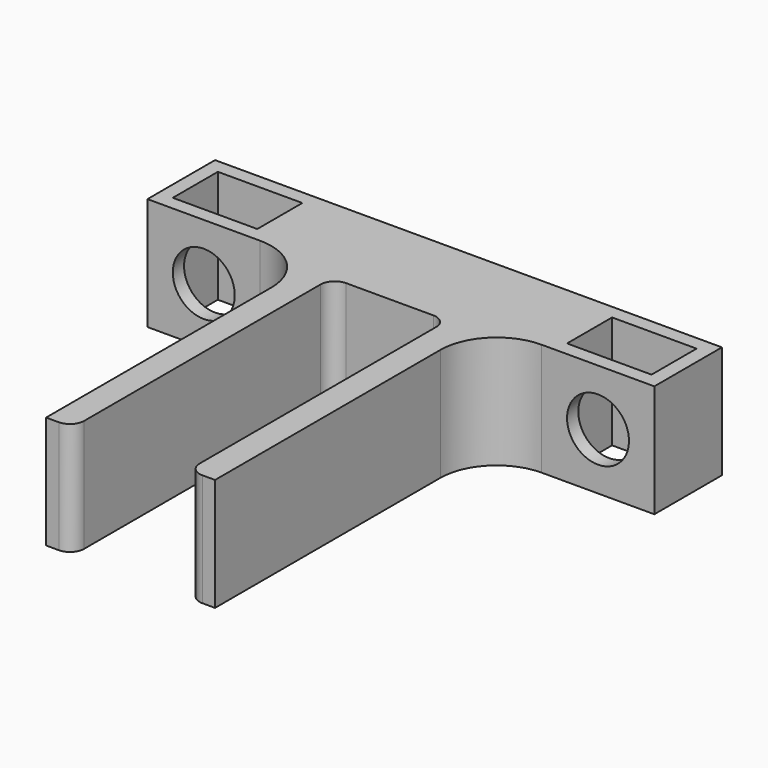
from build123d import *

# Parameters (mm, degrees)
F0_W         = 180
F0_H         = 40
F1_DEPTH     = 15
F2_W         = 60
F2_H         = 40
F3_DEPTH     = 120
F4_W         = 41
F4_H         = 40
F5_DEPTH     = 115
F6_R         = 20
F7_R         = 5
F8_TEXT_SIZE = 13.3061623071
F9_DEPTH     = 1
F10_W        = 30
F10_H        = 20
F11_DEPTH    = 40
F12_W        = 30
F12_H        = 20
F13_DEPTH    = 40
F15_D        = 22
F15_DEPTH    = 12
F15_TIP      = 6.6094668093
F17_D        = 22
F17_DEPTH    = 12
F17_TIP      = 6.6094668093


# Not quite as in the source:
# - Text() gives the source's letters only with a copy of the font that has no kerning and outlines rounded to 1/6400 em; it was checked with that copy


with BuildPart() as f1:
    # F0 (on Front) → F1 (new body, symmetric)
    with BuildSketch(Plane.XZ):
        with Locations((0, 6.5696623251)):
            Rectangle(F0_W, F0_H)
    extrude(amount=F1_DEPTH, both=True)

    # F2 (on face) → F3 (join)
    with BuildSketch(Plane.XZ.offset(15)):
        with Locations((0, 6.5696623251)):
            Rectangle(F2_W, F2_H)
    extrude(amount=F3_DEPTH)

    # F4 (on face) → F5 (cut)
    with BuildSketch(Plane.XZ.offset(135)):
        with Locations((0, 6.5696623251)):
            Rectangle(F4_W, F4_H)
    extrude(amount=-F5_DEPTH, mode=Mode.SUBTRACT)

    # F6
    f6_edges = [f1.edges().sort_by_distance(p)[0] for p in [
        (-30, -15, 6.569662),
        (30, -15, 6.569662),
    ]]
    fillet(f6_edges, radius=F6_R)

    # F7
    f7_edges = [f1.edges().sort_by_distance(p)[0] for p in [
        (-20.5, -20, 6.569662),
        (20.5, -20, 6.569662),
        (-20.5, -135, 6.569662),
        (20.5, -135, 6.569662),
    ]]
    fillet(f7_edges, radius=F7_R)

    # F8 (on face) → F9 (cut)
    with BuildSketch(Plane(origin=(0, 15, 0), x_dir=(-1, 0, 0), z_dir=(0, 1, 0))):
        with Locations((-20.5944048021, -9.5804368611)):
            Text('42mm', F8_TEXT_SIZE, font='Open Sans', font_style=FontStyle.BOLD, text_align=(TextAlign.LEFT, TextAlign.BOTTOM))
    extrude(amount=-F9_DEPTH, mode=Mode.SUBTRACT)

    # F10 (on face) → F11 (cut)
    with BuildSketch(Plane.XY.offset(26.5696623251)):
        with Locations((-70, 0)):
            Rectangle(F10_W, F10_H)
    extrude(amount=-F11_DEPTH, mode=Mode.SUBTRACT)

    # F12 (on face) → F13 (cut)
    with BuildSketch(Plane.XY.offset(26.5696623251)):
        with Locations((70, 0)):
            Rectangle(F12_W, F12_H)
    extrude(amount=-F13_DEPTH, mode=Mode.SUBTRACT)

    # F15
    with Locations(Plane.XZ.offset(15)):
        with Locations((-70, 6.5696623251)):
            Hole(F15_D / 2, depth=F15_DEPTH)
            with Locations((0, 0, -(F15_DEPTH + F15_TIP / 2))):  # 118° drill point
                Cone(0, F15_D / 2, F15_TIP, mode=Mode.SUBTRACT)

    # F17
    with Locations(Plane.XZ.offset(15)):
        with Locations((70, 6.5696623251)):
            Hole(F17_D / 2, depth=F17_DEPTH)
            with Locations((0, 0, -(F17_DEPTH + F17_TIP / 2))):  # 118° drill point
                Cone(0, F17_D / 2, F17_TIP, mode=Mode.SUBTRACT)


solid = f1.part
